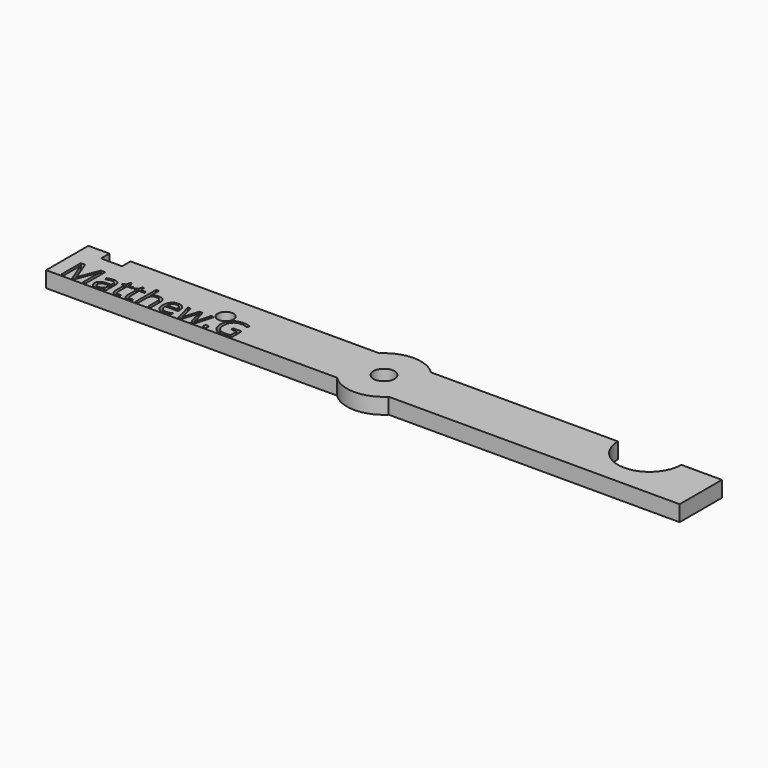
from build123d import *

# Parameters (mm, degrees)
F0_R         = 2
F0_R_2       = 1.5
F1_DEPTH     = 3
F2_TEXT_SIZE = 6.5259544903
F3_DEPTH     = 25


# Not quite as in the source:
# - Text() gives the source's letters only with a copy of the font that has no kerning and outlines rounded to 1/6400 em; it was checked with that copy


with BuildPart() as f1:
    # F0 (on Top) → F1 (new body)
    with BuildSketch(Plane.XY):
        with BuildLine():
            ThreePointArc((7, 0), (6.4534043883, -2.7117470016), (4.8989794856, -5))
            Line((4.8989794856, -5), (60, -5))
            Line((60, -5), (60, 5))
            Line((60, 5), (52.3093072176, 5))
            ThreePointArc((52.3093072176, 5), (46.3093072176, -1), (40.3093072176, 5))
            Line((40.3093072176, 5), (4.8989794856, 5))
            ThreePointArc((4.8989794856, 5), (6.4534043883, 2.7117470016), (7, 0))
        make_face()
        with BuildLine():
            ThreePointArc((-4.8989794856, 5), (-7, 0), (-4.8989794856, -5))
            Line((-4.8989794856, -5), (4.8989794856, -5))
            ThreePointArc((4.8989794856, -5), (6.4534043883, -2.7117470016), (7, 0))
            ThreePointArc((7, 0), (6.4534043883, 2.7117470016), (4.8989794856, 5))
            Line((4.8989794856, 5), (-4.8989794856, 5))
        make_face()
        Circle(F0_R, mode=Mode.SUBTRACT)
        with BuildLine():
            ThreePointArc((4.8989794856, 5), (0, 7), (-4.8989794856, 5))
            Line((-4.8989794856, 5), (4.8989794856, 5))
        make_face()
        with BuildLine():
            Line((4.8989794856, -5), (-4.8989794856, -5))
            ThreePointArc((-4.8989794856, -5), (0, -7), (4.8989794856, -5))
        make_face()
        with BuildLine():
            Line((-56, 5), (-60, 5))
            Line((-60, 5), (-60, -5))
            Line((-60, -5), (-4.8989794856, -5))
            ThreePointArc((-4.8989794856, -5), (-7, 0), (-4.8989794856, 5))
            Line((-4.8989794856, 5), (-52, 5))
            Line((-52, 5), (-52, 3))
            Line((-52, 3), (-56, 3))
            Line((-56, 3), (-56, 5))
        make_face()
        with Locations((-30, 0)):
            Circle(F0_R_2, mode=Mode.SUBTRACT)
    extrude(amount=F1_DEPTH)

    # F2 (on Top) → F3 (cut)
    with BuildSketch(Plane.XY):
        with Locations((-58.0375287682, -4.698687233)):
            Text('Matthew.G', F2_TEXT_SIZE, font='Open Sans', text_align=(TextAlign.LEFT, TextAlign.BOTTOM))
    extrude(amount=F3_DEPTH, mode=Mode.SUBTRACT)


solid = f1.part
